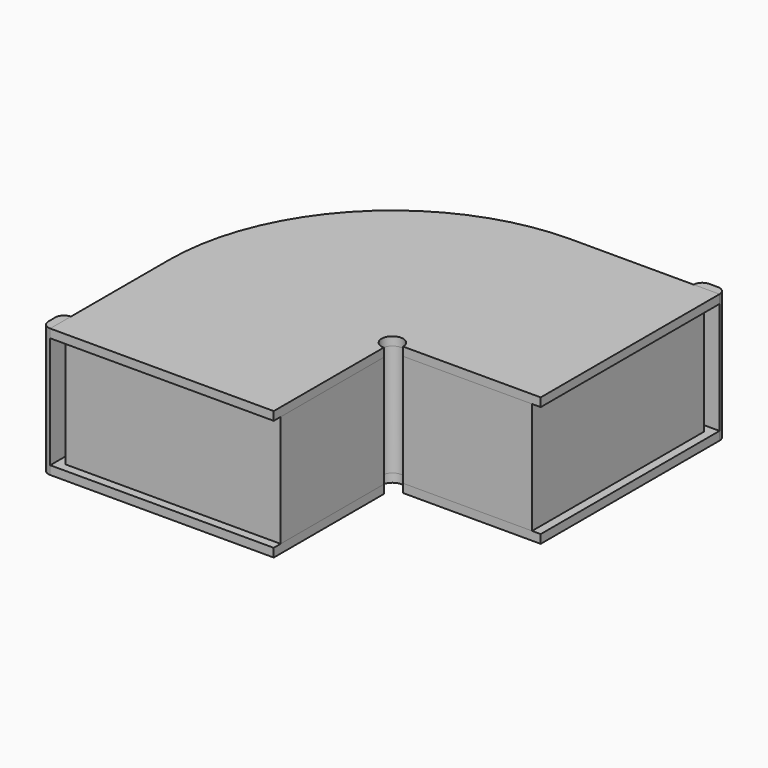
from build123d import *
from build123d import SkipClean  # not in build123d's __all__

# Parameters (mm, degrees)
F1_DEPTH = 26
F3_DEPTH = 2
F5_DEPTH = 2
F6_W     = 2
F6_H     = 6
F7_DEPTH = 30
F6_W_2   = 6
F6_H_2   = 2
F8_R     = 1.99999
F8_2_R   = 1.99999


# Not quite as in the source:
# - a fillet or chamfer is up to 0.001 mm smaller than in the source, because OpenCascade refuses the exact size


with BuildPart() as f1:
    # F0 (on Top) → F1 (new body)
    with BuildSketch(Plane.XY):
        with BuildLine():
            ThreePointArc((0, -2.5), (-1.767766953, 1.767766953), (2.5, 0))
            Line((2.5, 0), (32.5, 0))
            Line((32.5, 0), (32.5, 50))
            Line((32.5, 50), (0, 50))
            ThreePointArc((0, 50), (-35.3553390593, 35.3553390593), (-50, 0))
            Line((-50, 0), (-50, -32.5))
            Line((-50, -32.5), (0, -32.5))
            Line((0, -32.5), (0, -2.5))
        make_face()
    extrude(amount=F1_DEPTH)

    # F4 (on face) → F5 (join)
    with BuildSketch(Plane(origin=(0, 0, 0), x_dir=(1, 0, 0), z_dir=(0, 0, -1))):
        with BuildLine():
            Line((0, 34.5), (-52, 34.5))
            Line((-52, 34.5), (-52, 0))
            ThreePointArc((-52, 0), (-36.7695526217, -36.7695526217), (0, -52))
            Line((0, -52), (34.5, -52))
            Line((34.5, -52), (34.5, 0))
            Line((34.5, 0), (32.5, 0))
            Line((32.5, 0), (32.5, -50))
            Line((32.5, -50), (0, -50))
            ThreePointArc((0, -50), (-35.3553390593, -35.3553390593), (-50, 0))
            Line((-50, 0), (-50, 32.5))
            Line((-50, 32.5), (0, 32.5))
            Line((0, 32.5), (0, 34.5))
        make_face()
        with BuildLine():
            Line((0, 2.5), (0, 32.5))
            Line((0, 32.5), (-50, 32.5))
            Line((-50, 32.5), (-50, 0))
            ThreePointArc((-50, 0), (-35.3553390593, -35.3553390593), (0, -50))
            Line((0, -50), (32.5, -50))
            Line((32.5, -50), (32.5, 0))
            Line((32.5, 0), (2.5, 0))
            ThreePointArc((2.5, 0), (-1.767766953, -1.767766953), (0, 2.5))
        make_face()
    with SkipClean():  # cleaning this boolean's faces spoils the solid; the shape is the same uncleaned
        extrude(amount=F5_DEPTH)


with BuildPart() as f3:
    # F2 (on face) → F3 (new body)
    with BuildSketch(Plane.XY.offset(26)):
        with BuildLine():
            Line((34.5, 0), (34.5, 52))
            Line((34.5, 52), (0, 52))
            ThreePointArc((0, 52), (-36.7695526217, 36.7695526217), (-52, 0))
            Line((-52, 0), (-52, -34.5))
            Line((-52, -34.5), (0, -34.5))
            Line((0, -34.5), (0, -32.5))
            Line((0, -32.5), (-50, -32.5))
            Line((-50, -32.5), (-50, 0))
            ThreePointArc((-50, 0), (-35.3553390593, 35.3553390593), (0, 50))
            Line((0, 50), (32.5, 50))
            Line((32.5, 50), (32.5, 0))
            Line((32.5, 0), (34.5, 0))
        make_face()
        with BuildLine():
            Line((2.5, 0), (32.5, 0))
            Line((32.5, 0), (32.5, 50))
            Line((32.5, 50), (0, 50))
            ThreePointArc((0, 50), (-35.3553390593, 35.3553390593), (-50, 0))
            Line((-50, 0), (-50, -32.5))
            Line((-50, -32.5), (0, -32.5))
            Line((0, -32.5), (0, -2.5))
            ThreePointArc((0, -2.5), (-1.767766953, 1.767766953), (2.5, 0))
        make_face()
    extrude(amount=F3_DEPTH)


with BuildPart() as f7:
    # F6 (on face) → F7 (new body, through all)
    with BuildSketch(Plane.XY.offset(28)):
        with Locations((-53, -31.5)):
            Rectangle(F6_W, F6_H)
    extrude(amount=-F7_DEPTH)

    # F8#2 (radius 2 in the source; OpenCascade refuses exactly that, so slightly less here)
    f8_2_edges = [f7.edges().sort_by_distance(p)[0] for p in [
        (-54, -28.5, 13),
        (-54, -34.5, 13),
    ]]
    fillet(f8_2_edges, radius=F8_2_R)


with BuildPart() as f7b:
    # F6 (on face) → F7, piece 2 (new body, through all)
    with BuildSketch(Plane.XY.offset(28)):
        with Locations((31.5, 53)):
            Rectangle(F6_W_2, F6_H_2)
    extrude(amount=-F7_DEPTH)

    # F8 (radius 2 in the source; OpenCascade refuses exactly that, so slightly less here)
    f8_edges = [f7b.edges().sort_by_distance(p)[0] for p in [
        (28.5, 54, 13),
        (34.5, 54, 13),
    ]]
    fillet(f8_edges, radius=F8_R)


solid = Compound([f1.part, f3.part, f7.part, f7b.part])
